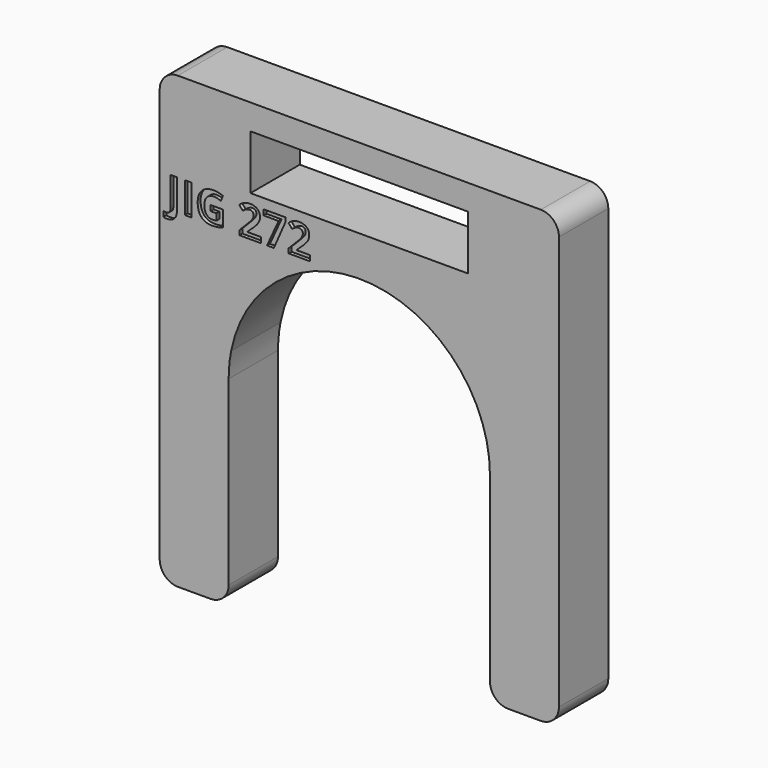
from build123d import *

# Parameters (mm, degrees)
F0_W     = 1.204434487
F0_H     = 8.486159523
F0_W_2   = 0.5953222601
F1_DEPTH = 17
F2_DEPTH = 5
F3_R     = 5
F4_DEPTH = 19
F5_DEPTH = 3


# Not quite as in the source:
# - a feature names something its author has since deleted; it is built from what else it names


with BuildPart() as f1:
    # F0 (on Front) → F1 (new body)
    with BuildSketch(Plane.XZ):
        with BuildLine():
            Line((0, 40), (0, 29))
            ThreePointArc((0, 29), (25.4558441227, 18.4558441227), (36, -7))
            Line((36, -7), (36, -62))
            Line((36, -62), (47.5, -62))
            Line((47.5, -62), (55, -62))
            Line((55, -62), (55, 0))
            Line((55, 0), (55, 62))
            Line((55, 62), (0, 62))
            Line((0, 62), (0, 55))
            Line((0, 55), (30, 55))
            Line((30, 55), (30, 40))
            Line((30, 40), (0, 40))
        make_face()
        with BuildLine():
            ThreePointArc((51, -33), (49.9748737342, -35.4748737342), (47.5, -36.5))
            ThreePointArc((47.5, -36.5), (44, -33), (47.5, -29.5))
            ThreePointArc((47.5, -29.5), (49.9748737342, -30.5251262658), (51, -33))
        make_face(mode=Mode.SUBTRACT)
        with BuildLine():
            ThreePointArc((50.5, 55), (49.6213203436, 52.8786796564), (47.5, 52))
            ThreePointArc((47.5, 52), (45.3786796564, 57.1213203436), (50.5, 55))
        make_face(mode=Mode.SUBTRACT)
        with BuildLine():
            Line((-36, 0), (-35.312887166, 0))
            ThreePointArc((-35.312887166, 0), (-22.8473193176, 20.8208554865), (0, 29))
            Line((0, 29), (0, 40))
            Line((0, 40), (-30, 40))
            Line((-30, 40), (-30, 55))
            Line((-30, 55), (0, 55))
            Line((0, 55), (0, 62))
            Line((0, 62), (-55, 62))
            Line((-55, 62), (-55, 0))
            Line((-55, 0), (-47.5, 0))
            Line((-47.5, 0), (-36, 0))
        make_face()
        with BuildLine():
            add(Edge.make_bspline(
                [(-50.9101120954, 27.0733917031), (-51.5889677105, 26.2951687134), (-52.9188189293, 26.2951687134)],
                knots=[0, 0, 0, 1, 1, 1], degree=2))
            add(Edge.make_bspline(
                [(-52.9188189293, 26.2951687134), (-53.5280245155, 26.2951687134), (-53.981214037, 26.4233247666)],
                knots=[0, 0, 0, 1, 1, 1], degree=2))
            Line((-53.981214037, 26.4233247666), (-53.981214037, 27.9203360547))
            add(Edge.make_bspline(
                [(-53.981214037, 27.9203360547), (-53.5168805109, 27.8051813402), (-53.1342696854, 27.8051813402)],
                knots=[0, 0, 0, 1, 1, 1], degree=2))
            add(Edge.make_bspline(
                [(-53.1342696854, 27.8051813402), (-52.5417801061, 27.8051813402), (-52.2863966667, 28.1738621599)],
                knots=[0, 0, 0, 1, 1, 1], degree=2))
            add(Edge.make_bspline(
                [(-52.2863966667, 28.1738621599), (-52.0310132274, 28.5425429797), (-52.0310132274, 29.3263379717)],
                knots=[0, 0, 0, 1, 1, 1], degree=2))
            Line((-52.0310132274, 29.3263379717), (-52.0310132274, 37.2775852726))
            Line((-52.0310132274, 37.2775852726), (-50.2312564802, 37.2775852726))
            Line((-50.2312564802, 37.2775852726), (-50.2312564802, 29.3374819764))
            add(Edge.make_bspline(
                [(-50.2312564802, 29.3374819764), (-50.2312564802, 27.8516146928), (-50.9101120954, 27.0733917031)],
                knots=[0, 0, 0, 1, 1, 1], degree=2))
        make_face(mode=Mode.SUBTRACT)
        Polygon((-46.295565513, 28.7914257497), (-47.5, 28.7914257497), (-48.0953222601, 28.7914257497), (-48.0953222601, 37.2775852726), (-47.5, 37.2775852726), (-46.295565513, 37.2775852726), align=None, mode=Mode.SUBTRACT)
        with BuildLine():
            Line((-40.9390139559, 32.0584764393), (-40.9390139559, 33.5573450615))
            Line((-40.9390139559, 33.5573450615), (-37.5716672247, 33.5573450615))
            Line((-37.5716672247, 33.5573450615), (-37.5716672247, 29.1573205682))
            add(Edge.make_bspline(
                [(-37.5716672247, 29.1573205682), (-38.3907515647, 28.8898644572), (-39.1132545313, 28.7821390791)],
                knots=[0, 0, 0, 1, 1, 1], degree=2))
            add(Edge.make_bspline(
                [(-39.1132545313, 28.7821390791), (-39.8357574979, 28.6744137011), (-40.5898351443, 28.6744137011)],
                knots=[0, 0, 0, 1, 1, 1], degree=2))
            add(Edge.make_bspline(
                [(-40.5898351443, 28.6744137011), (-42.5103186082, 28.6744137011), (-43.5234943622, 29.8036728366)],
                knots=[0, 0, 0, 1, 1, 1], degree=2))
            add(Edge.make_bspline(
                [(-43.5234943622, 29.8036728366), (-44.5366701161, 30.932931972), (-44.5366701161, 33.0465781828)],
                knots=[0, 0, 0, 1, 1, 1], degree=2))
            add(Edge.make_bspline(
                [(-44.5366701161, 33.0465781828), (-44.5366701161, 35.1007897023), (-43.3609776281, 36.2495508458)],
                knots=[0, 0, 0, 1, 1, 1], degree=2))
            add(Edge.make_bspline(
                [(-43.3609776281, 36.2495508458), (-42.18528514, 37.3983119894), (-40.1032136089, 37.3983119894)],
                knots=[0, 0, 0, 1, 1, 1], degree=2))
            add(Edge.make_bspline(
                [(-40.1032136089, 37.3983119894), (-38.7956503995, 37.3983119894), (-37.5828112293, 36.8764011061)],
                knots=[0, 0, 0, 1, 1, 1], degree=2))
            Line((-37.5828112293, 36.8764011061), (-38.1808728109, 35.4369671752))
            add(Edge.make_bspline(
                [(-38.1808728109, 35.4369671752), (-39.1095398631, 35.9013007013), (-40.1143576136, 35.9013007013)],
                knots=[0, 0, 0, 1, 1, 1], degree=2))
            add(Edge.make_bspline(
                [(-40.1143576136, 35.9013007013), (-41.2807634311, 35.9013007013), (-41.9828357226, 35.1175057092)],
                knots=[0, 0, 0, 1, 1, 1], degree=2))
            add(Edge.make_bspline(
                [(-41.9828357226, 35.1175057092), (-42.6849080141, 34.3337107172), (-42.6849080141, 33.0112888348)],
                knots=[0, 0, 0, 1, 1, 1], degree=2))
            add(Edge.make_bspline(
                [(-42.6849080141, 33.0112888348), (-42.6849080141, 31.6294322612), (-42.1193497793, 30.9013572922)],
                knots=[0, 0, 0, 1, 1, 1], degree=2))
            add(Edge.make_bspline(
                [(-42.1193497793, 30.9013572922), (-41.5537915445, 30.1732823233), (-40.4746804298, 30.1732823233)],
                knots=[0, 0, 0, 1, 1, 1], degree=2))
            add(Edge.make_bspline(
                [(-40.4746804298, 30.1732823233), (-39.9100508621, 30.1732823233), (-39.3305626215, 30.2884370378)],
                knots=[0, 0, 0, 1, 1, 1], degree=2))
            Line((-39.3305626215, 30.2884370378), (-39.3305626215, 32.0584764393))
            Line((-39.3305626215, 32.0584764393), (-40.9390139559, 32.0584764393))
        make_face(mode=Mode.SUBTRACT)
        with BuildLine():
            Line((-27.1241628875, 30.3014383765), (-27.1241628875, 28.7914257497))
            Line((-27.1241628875, 28.7914257497), (-33.0564880169, 28.7914257497))
            Line((-33.0564880169, 28.7914257497), (-33.0564880169, 30.0395542678))
            Line((-33.0564880169, 30.0395542678), (-30.9261257991, 32.1922044948))
            add(Edge.make_bspline(
                [(-30.9261257991, 32.1922044948), (-29.9788854059, 33.1617328973), (-29.6891412856, 33.5359857193)],
                knots=[0, 0, 0, 1, 1, 1], degree=2))
            add(Edge.make_bspline(
                [(-29.6891412856, 33.5359857193), (-29.3993971653, 33.9102385414), (-29.2712411121, 34.2297000073)],
                knots=[0, 0, 0, 1, 1, 1], degree=2))
            add(Edge.make_bspline(
                [(-29.2712411121, 34.2297000073), (-29.1430850589, 34.5491614733), (-29.1430850589, 34.8909109485)],
                knots=[0, 0, 0, 1, 1, 1], degree=2))
            add(Edge.make_bspline(
                [(-29.1430850589, 34.8909109485), (-29.1430850589, 35.4016778272), (-29.4253998428, 35.6514892642)],
                knots=[0, 0, 0, 1, 1, 1], degree=2))
            add(Edge.make_bspline(
                [(-29.4253998428, 35.6514892642), (-29.7077146267, 35.9013007013), (-30.1776201551, 35.9013007013)],
                knots=[0, 0, 0, 1, 1, 1], degree=2))
            add(Edge.make_bspline(
                [(-30.1776201551, 35.9013007013), (-30.6698136927, 35.9013007013), (-31.1341472188, 35.6747059405)],
                knots=[0, 0, 0, 1, 1, 1], degree=2))
            add(Edge.make_bspline(
                [(-31.1341472188, 35.6747059405), (-31.5984807449, 35.4481111798), (-32.1036756213, 35.0302110063)],
                knots=[0, 0, 0, 1, 1, 1], degree=2))
            Line((-32.1036756213, 35.0302110063), (-33.0787760261, 36.1854728192))
            add(Edge.make_bspline(
                [(-33.0787760261, 36.1854728192), (-32.452854433, 36.7203850413), (-32.0405262618, 36.9404791327)],
                knots=[0, 0, 0, 1, 1, 1], degree=2))
            add(Edge.make_bspline(
                [(-32.0405262618, 36.9404791327), (-31.6281980906, 37.1605732241), (-31.1406478882, 37.2794426067)],
                knots=[0, 0, 0, 1, 1, 1], degree=2))
            add(Edge.make_bspline(
                [(-31.1406478882, 37.2794426067), (-30.6530976858, 37.3983119894), (-30.0494641019, 37.3983119894)],
                knots=[0, 0, 0, 1, 1, 1], degree=2))
            add(Edge.make_bspline(
                [(-30.0494641019, 37.3983119894), (-29.2545251052, 37.3983119894), (-28.645319519, 37.1085678691)],
                knots=[0, 0, 0, 1, 1, 1], degree=2))
            add(Edge.make_bspline(
                [(-28.645319519, 37.1085678691), (-28.0361139327, 36.8188237488), (-27.6990077928, 36.2959841985)],
                knots=[0, 0, 0, 1, 1, 1], degree=2))
            add(Edge.make_bspline(
                [(-27.6990077928, 36.2959841985), (-27.3619016528, 35.7731446481), (-27.3619016528, 35.1007897023)],
                knots=[0, 0, 0, 1, 1, 1], degree=2))
            add(Edge.make_bspline(
                [(-27.3619016528, 35.1007897023), (-27.3619016528, 34.5138721253), (-27.5680657384, 34.0003192454)],
                knots=[0, 0, 0, 1, 1, 1], degree=2))
            add(Edge.make_bspline(
                [(-27.5680657384, 34.0003192454), (-27.774229824, 33.4867663656), (-28.2069886703, 32.9472108082)],
                knots=[0, 0, 0, 1, 1, 1], degree=2))
            add(Edge.make_bspline(
                [(-28.2069886703, 32.9472108082), (-28.6397475166, 32.4076552509), (-29.7300026359, 31.4084095027)],
                knots=[0, 0, 0, 1, 1, 1], degree=2))
            Line((-29.7300026359, 31.4084095027), (-30.8221150893, 30.381303743))
            Line((-30.8221150893, 30.381303743), (-30.8221150893, 30.3014383765))
            Line((-30.8221150893, 30.3014383765), (-27.1241628875, 30.3014383765))
        make_face(mode=Mode.SUBTRACT)
        with BuildLine():
            ThreePointArc((-44.5, 55), (-45.3786796564, 52.8786796564), (-47.5, 52))
            ThreePointArc((-47.5, 52), (-49.6213203436, 57.1213203436), (-44.5, 55))
        make_face(mode=Mode.SUBTRACT)
        Polygon((-23.5487947365, 28.7914257497), (-25.4302741842, 28.7914257497), (-22.2430888611, 35.7564286411), (-26.4276625983, 35.7564286411), (-26.4276625983, 37.266441268), (-20.3393214041, 37.266441268), (-20.3393214041, 36.1390394666), align=None, mode=Mode.SUBTRACT)
        with BuildLine():
            Line((-13.5544799208, 30.3014383765), (-13.5544799208, 28.7914257497))
            Line((-13.5544799208, 28.7914257497), (-19.4868050502, 28.7914257497))
            Line((-19.4868050502, 28.7914257497), (-19.4868050502, 30.0395542678))
            Line((-19.4868050502, 30.0395542678), (-17.3564428325, 32.1922044948))
            add(Edge.make_bspline(
                [(-17.3564428325, 32.1922044948), (-16.4092024392, 33.1617328973), (-16.1194583189, 33.5359857193)],
                knots=[0, 0, 0, 1, 1, 1], degree=2))
            add(Edge.make_bspline(
                [(-16.1194583189, 33.5359857193), (-15.8297141986, 33.9102385414), (-15.7015581454, 34.2297000073)],
                knots=[0, 0, 0, 1, 1, 1], degree=2))
            add(Edge.make_bspline(
                [(-15.7015581454, 34.2297000073), (-15.5734020922, 34.5491614733), (-15.5734020922, 34.8909109485)],
                knots=[0, 0, 0, 1, 1, 1], degree=2))
            add(Edge.make_bspline(
                [(-15.5734020922, 34.8909109485), (-15.5734020922, 35.4016778272), (-15.8557168761, 35.6514892642)],
                knots=[0, 0, 0, 1, 1, 1], degree=2))
            add(Edge.make_bspline(
                [(-15.8557168761, 35.6514892642), (-16.13803166, 35.9013007013), (-16.6079371884, 35.9013007013)],
                knots=[0, 0, 0, 1, 1, 1], degree=2))
            add(Edge.make_bspline(
                [(-16.6079371884, 35.9013007013), (-17.100130726, 35.9013007013), (-17.5644642521, 35.6747059405)],
                knots=[0, 0, 0, 1, 1, 1], degree=2))
            add(Edge.make_bspline(
                [(-17.5644642521, 35.6747059405), (-18.0287977782, 35.4481111798), (-18.5339926546, 35.0302110063)],
                knots=[0, 0, 0, 1, 1, 1], degree=2))
            Line((-18.5339926546, 35.0302110063), (-19.5090930594, 36.1854728192))
            add(Edge.make_bspline(
                [(-19.5090930594, 36.1854728192), (-18.8831714663, 36.7203850413), (-18.4708432951, 36.9404791327)],
                knots=[0, 0, 0, 1, 1, 1], degree=2))
            add(Edge.make_bspline(
                [(-18.4708432951, 36.9404791327), (-18.0585151239, 37.1605732241), (-17.5709649215, 37.2794426067)],
                knots=[0, 0, 0, 1, 1, 1], degree=2))
            add(Edge.make_bspline(
                [(-17.5709649215, 37.2794426067), (-17.0834147191, 37.3983119894), (-16.4797811352, 37.3983119894)],
                knots=[0, 0, 0, 1, 1, 1], degree=2))
            add(Edge.make_bspline(
                [(-16.4797811352, 37.3983119894), (-15.6848421385, 37.3983119894), (-15.0756365523, 37.1085678691)],
                knots=[0, 0, 0, 1, 1, 1], degree=2))
            add(Edge.make_bspline(
                [(-15.0756365523, 37.1085678691), (-14.466430966, 36.8188237488), (-14.1293248261, 36.2959841985)],
                knots=[0, 0, 0, 1, 1, 1], degree=2))
            add(Edge.make_bspline(
                [(-14.1293248261, 36.2959841985), (-13.7922186861, 35.7731446481), (-13.7922186861, 35.1007897023)],
                knots=[0, 0, 0, 1, 1, 1], degree=2))
            add(Edge.make_bspline(
                [(-13.7922186861, 35.1007897023), (-13.7922186861, 34.5138721253), (-13.9983827717, 34.0003192454)],
                knots=[0, 0, 0, 1, 1, 1], degree=2))
            add(Edge.make_bspline(
                [(-13.9983827717, 34.0003192454), (-14.2045468573, 33.4867663656), (-14.6373057036, 32.9472108082)],
                knots=[0, 0, 0, 1, 1, 1], degree=2))
            add(Edge.make_bspline(
                [(-14.6373057036, 32.9472108082), (-15.0700645499, 32.4076552509), (-16.1603196692, 31.4084095027)],
                knots=[0, 0, 0, 1, 1, 1], degree=2))
            Line((-16.1603196692, 31.4084095027), (-17.2524321226, 30.381303743))
            Line((-17.2524321226, 30.381303743), (-17.2524321226, 30.3014383765))
            Line((-17.2524321226, 30.3014383765), (-13.5544799208, 30.3014383765))
        make_face(mode=Mode.SUBTRACT)
        with BuildLine():
            Line((-36, -7), (-36, 0))
            Line((-36, 0), (-47.5, 0))
            Line((-47.5, 0), (-47.5, -29.5))
            ThreePointArc((-47.5, -29.5), (-45.0251262658, -30.5251262658), (-44, -33))
            ThreePointArc((-44, -33), (-45.0251262658, -35.4748737342), (-47.5, -36.5))
            Line((-47.5, -36.5), (-47.5, -62))
            Line((-47.5, -62), (-36, -62))
            Line((-36, -62), (-36, -7))
        make_face()
        with BuildLine():
            Line((-47.5, -29.5), (-47.5, 0))
            Line((-47.5, 0), (-55, 0))
            Line((-55, 0), (-55, -62))
            Line((-55, -62), (-47.5, -62))
            Line((-47.5, -62), (-47.5, -36.5))
            ThreePointArc((-47.5, -36.5), (-51, -33), (-47.5, -29.5))
        make_face()
        with BuildLine():
            Line((-37.5716672247, 33.5573450615), (-40.9390139559, 33.5573450615))
            Line((-40.9390139559, 33.5573450615), (-40.9390139559, 32.0584764393))
            Line((-40.9390139559, 32.0584764393), (-39.3305626215, 32.0584764393))
            Line((-39.3305626215, 32.0584764393), (-39.3305626215, 30.2884370378))
            add(Edge.make_bspline(
                [(-40.4746804298, 30.1732823233), (-39.9100508621, 30.1732823233), (-39.3305626215, 30.2884370378)],
                knots=[0, 0, 0, 1, 1, 1], degree=2))
            add(Edge.make_bspline(
                [(-42.1193497793, 30.9013572922), (-41.5537915445, 30.1732823233), (-40.4746804298, 30.1732823233)],
                knots=[0, 0, 0, 1, 1, 1], degree=2))
            add(Edge.make_bspline(
                [(-42.6849080141, 33.0112888348), (-42.6849080141, 31.6294322612), (-42.1193497793, 30.9013572922)],
                knots=[0, 0, 0, 1, 1, 1], degree=2))
            add(Edge.make_bspline(
                [(-41.9828357226, 35.1175057092), (-42.6849080141, 34.3337107172), (-42.6849080141, 33.0112888348)],
                knots=[0, 0, 0, 1, 1, 1], degree=2))
            add(Edge.make_bspline(
                [(-40.1143576136, 35.9013007013), (-41.2807634311, 35.9013007013), (-41.9828357226, 35.1175057092)],
                knots=[0, 0, 0, 1, 1, 1], degree=2))
            add(Edge.make_bspline(
                [(-38.1808728109, 35.4369671752), (-39.1095398631, 35.9013007013), (-40.1143576136, 35.9013007013)],
                knots=[0, 0, 0, 1, 1, 1], degree=2))
            Line((-38.1808728109, 35.4369671752), (-37.5828112293, 36.8764011061))
            add(Edge.make_bspline(
                [(-40.1032136089, 37.3983119894), (-38.7956503995, 37.3983119894), (-37.5828112293, 36.8764011061)],
                knots=[0, 0, 0, 1, 1, 1], degree=2))
            add(Edge.make_bspline(
                [(-43.3609776281, 36.2495508458), (-42.18528514, 37.3983119894), (-40.1032136089, 37.3983119894)],
                knots=[0, 0, 0, 1, 1, 1], degree=2))
            add(Edge.make_bspline(
                [(-44.5366701161, 33.0465781828), (-44.5366701161, 35.1007897023), (-43.3609776281, 36.2495508458)],
                knots=[0, 0, 0, 1, 1, 1], degree=2))
            add(Edge.make_bspline(
                [(-43.5234943622, 29.8036728366), (-44.5366701161, 30.932931972), (-44.5366701161, 33.0465781828)],
                knots=[0, 0, 0, 1, 1, 1], degree=2))
            add(Edge.make_bspline(
                [(-40.5898351443, 28.6744137011), (-42.5103186082, 28.6744137011), (-43.5234943622, 29.8036728366)],
                knots=[0, 0, 0, 1, 1, 1], degree=2))
            add(Edge.make_bspline(
                [(-39.1132545313, 28.7821390791), (-39.8357574979, 28.6744137011), (-40.5898351443, 28.6744137011)],
                knots=[0, 0, 0, 1, 1, 1], degree=2))
            add(Edge.make_bspline(
                [(-37.5716672247, 29.1573205682), (-38.3907515647, 28.8898644572), (-39.1132545313, 28.7821390791)],
                knots=[0, 0, 0, 1, 1, 1], degree=2))
            Line((-37.5716672247, 29.1573205682), (-37.5716672247, 33.5573450615))
        make_face()
        with BuildLine():
            ThreePointArc((-44.5, 55), (-49.6213203436, 57.1213203436), (-47.5, 52))
            ThreePointArc((-47.5, 52), (-45.3786796564, 52.8786796564), (-44.5, 55))
        make_face()
        with BuildLine():
            ThreePointArc((50.5, 55), (45.3786796564, 57.1213203436), (47.5, 52))
            ThreePointArc((47.5, 52), (49.6213203436, 52.8786796564), (50.5, 55))
        make_face()
        with BuildLine():
            Line((-33.0564880169, 28.7914257497), (-27.1241628875, 28.7914257497))
            Line((-27.1241628875, 28.7914257497), (-27.1241628875, 30.3014383765))
            Line((-27.1241628875, 30.3014383765), (-30.8221150893, 30.3014383765))
            Line((-30.8221150893, 30.3014383765), (-30.8221150893, 30.381303743))
            Line((-30.8221150893, 30.381303743), (-29.7300026359, 31.4084095027))
            add(Edge.make_bspline(
                [(-28.2069886703, 32.9472108082), (-28.6397475166, 32.4076552509), (-29.7300026359, 31.4084095027)],
                knots=[0, 0, 0, 1, 1, 1], degree=2))
            add(Edge.make_bspline(
                [(-27.5680657384, 34.0003192454), (-27.774229824, 33.4867663656), (-28.2069886703, 32.9472108082)],
                knots=[0, 0, 0, 1, 1, 1], degree=2))
            add(Edge.make_bspline(
                [(-27.3619016528, 35.1007897023), (-27.3619016528, 34.5138721253), (-27.5680657384, 34.0003192454)],
                knots=[0, 0, 0, 1, 1, 1], degree=2))
            add(Edge.make_bspline(
                [(-27.6990077928, 36.2959841985), (-27.3619016528, 35.7731446481), (-27.3619016528, 35.1007897023)],
                knots=[0, 0, 0, 1, 1, 1], degree=2))
            add(Edge.make_bspline(
                [(-28.645319519, 37.1085678691), (-28.0361139327, 36.8188237488), (-27.6990077928, 36.2959841985)],
                knots=[0, 0, 0, 1, 1, 1], degree=2))
            add(Edge.make_bspline(
                [(-30.0494641019, 37.3983119894), (-29.2545251052, 37.3983119894), (-28.645319519, 37.1085678691)],
                knots=[0, 0, 0, 1, 1, 1], degree=2))
            add(Edge.make_bspline(
                [(-31.1406478882, 37.2794426067), (-30.6530976858, 37.3983119894), (-30.0494641019, 37.3983119894)],
                knots=[0, 0, 0, 1, 1, 1], degree=2))
            add(Edge.make_bspline(
                [(-32.0405262618, 36.9404791327), (-31.6281980906, 37.1605732241), (-31.1406478882, 37.2794426067)],
                knots=[0, 0, 0, 1, 1, 1], degree=2))
            add(Edge.make_bspline(
                [(-33.0787760261, 36.1854728192), (-32.452854433, 36.7203850413), (-32.0405262618, 36.9404791327)],
                knots=[0, 0, 0, 1, 1, 1], degree=2))
            Line((-33.0787760261, 36.1854728192), (-32.1036756213, 35.0302110063))
            add(Edge.make_bspline(
                [(-31.1341472188, 35.6747059405), (-31.5984807449, 35.4481111798), (-32.1036756213, 35.0302110063)],
                knots=[0, 0, 0, 1, 1, 1], degree=2))
            add(Edge.make_bspline(
                [(-30.1776201551, 35.9013007013), (-30.6698136927, 35.9013007013), (-31.1341472188, 35.6747059405)],
                knots=[0, 0, 0, 1, 1, 1], degree=2))
            add(Edge.make_bspline(
                [(-29.4253998428, 35.6514892642), (-29.7077146267, 35.9013007013), (-30.1776201551, 35.9013007013)],
                knots=[0, 0, 0, 1, 1, 1], degree=2))
            add(Edge.make_bspline(
                [(-29.1430850589, 34.8909109485), (-29.1430850589, 35.4016778272), (-29.4253998428, 35.6514892642)],
                knots=[0, 0, 0, 1, 1, 1], degree=2))
            add(Edge.make_bspline(
                [(-29.2712411121, 34.2297000073), (-29.1430850589, 34.5491614733), (-29.1430850589, 34.8909109485)],
                knots=[0, 0, 0, 1, 1, 1], degree=2))
            add(Edge.make_bspline(
                [(-29.6891412856, 33.5359857193), (-29.3993971653, 33.9102385414), (-29.2712411121, 34.2297000073)],
                knots=[0, 0, 0, 1, 1, 1], degree=2))
            add(Edge.make_bspline(
                [(-30.9261257991, 32.1922044948), (-29.9788854059, 33.1617328973), (-29.6891412856, 33.5359857193)],
                knots=[0, 0, 0, 1, 1, 1], degree=2))
            Line((-30.9261257991, 32.1922044948), (-33.0564880169, 30.0395542678))
            Line((-33.0564880169, 30.0395542678), (-33.0564880169, 28.7914257497))
        make_face()
        with BuildLine():
            Line((-19.4868050502, 28.7914257497), (-13.5544799208, 28.7914257497))
            Line((-13.5544799208, 28.7914257497), (-13.5544799208, 30.3014383765))
            Line((-13.5544799208, 30.3014383765), (-17.2524321226, 30.3014383765))
            Line((-17.2524321226, 30.3014383765), (-17.2524321226, 30.381303743))
            Line((-17.2524321226, 30.381303743), (-16.1603196692, 31.4084095027))
            add(Edge.make_bspline(
                [(-14.6373057036, 32.9472108082), (-15.0700645499, 32.4076552509), (-16.1603196692, 31.4084095027)],
                knots=[0, 0, 0, 1, 1, 1], degree=2))
            add(Edge.make_bspline(
                [(-13.9983827717, 34.0003192454), (-14.2045468573, 33.4867663656), (-14.6373057036, 32.9472108082)],
                knots=[0, 0, 0, 1, 1, 1], degree=2))
            add(Edge.make_bspline(
                [(-13.7922186861, 35.1007897023), (-13.7922186861, 34.5138721253), (-13.9983827717, 34.0003192454)],
                knots=[0, 0, 0, 1, 1, 1], degree=2))
            add(Edge.make_bspline(
                [(-14.1293248261, 36.2959841985), (-13.7922186861, 35.7731446481), (-13.7922186861, 35.1007897023)],
                knots=[0, 0, 0, 1, 1, 1], degree=2))
            add(Edge.make_bspline(
                [(-15.0756365523, 37.1085678691), (-14.466430966, 36.8188237488), (-14.1293248261, 36.2959841985)],
                knots=[0, 0, 0, 1, 1, 1], degree=2))
            add(Edge.make_bspline(
                [(-16.4797811352, 37.3983119894), (-15.6848421385, 37.3983119894), (-15.0756365523, 37.1085678691)],
                knots=[0, 0, 0, 1, 1, 1], degree=2))
            add(Edge.make_bspline(
                [(-17.5709649215, 37.2794426067), (-17.0834147191, 37.3983119894), (-16.4797811352, 37.3983119894)],
                knots=[0, 0, 0, 1, 1, 1], degree=2))
            add(Edge.make_bspline(
                [(-18.4708432951, 36.9404791327), (-18.0585151239, 37.1605732241), (-17.5709649215, 37.2794426067)],
                knots=[0, 0, 0, 1, 1, 1], degree=2))
            add(Edge.make_bspline(
                [(-19.5090930594, 36.1854728192), (-18.8831714663, 36.7203850413), (-18.4708432951, 36.9404791327)],
                knots=[0, 0, 0, 1, 1, 1], degree=2))
            Line((-19.5090930594, 36.1854728192), (-18.5339926546, 35.0302110063))
            add(Edge.make_bspline(
                [(-17.5644642521, 35.6747059405), (-18.0287977782, 35.4481111798), (-18.5339926546, 35.0302110063)],
                knots=[0, 0, 0, 1, 1, 1], degree=2))
            add(Edge.make_bspline(
                [(-16.6079371884, 35.9013007013), (-17.100130726, 35.9013007013), (-17.5644642521, 35.6747059405)],
                knots=[0, 0, 0, 1, 1, 1], degree=2))
            add(Edge.make_bspline(
                [(-15.8557168761, 35.6514892642), (-16.13803166, 35.9013007013), (-16.6079371884, 35.9013007013)],
                knots=[0, 0, 0, 1, 1, 1], degree=2))
            add(Edge.make_bspline(
                [(-15.5734020922, 34.8909109485), (-15.5734020922, 35.4016778272), (-15.8557168761, 35.6514892642)],
                knots=[0, 0, 0, 1, 1, 1], degree=2))
            add(Edge.make_bspline(
                [(-15.7015581454, 34.2297000073), (-15.5734020922, 34.5491614733), (-15.5734020922, 34.8909109485)],
                knots=[0, 0, 0, 1, 1, 1], degree=2))
            add(Edge.make_bspline(
                [(-16.1194583189, 33.5359857193), (-15.8297141986, 33.9102385414), (-15.7015581454, 34.2297000073)],
                knots=[0, 0, 0, 1, 1, 1], degree=2))
            add(Edge.make_bspline(
                [(-17.3564428325, 32.1922044948), (-16.4092024392, 33.1617328973), (-16.1194583189, 33.5359857193)],
                knots=[0, 0, 0, 1, 1, 1], degree=2))
            Line((-17.3564428325, 32.1922044948), (-19.4868050502, 30.0395542678))
            Line((-19.4868050502, 30.0395542678), (-19.4868050502, 28.7914257497))
        make_face()
        Polygon((-22.2430888611, 35.7564286411), (-25.4302741842, 28.7914257497), (-23.5487947365, 28.7914257497), (-20.3393214041, 36.1390394666), (-20.3393214041, 37.266441268), (-26.4276625983, 37.266441268), (-26.4276625983, 35.7564286411), align=None)
        with BuildLine():
            add(Edge.make_bspline(
                [(-52.9188189293, 26.2951687134), (-53.5280245155, 26.2951687134), (-53.981214037, 26.4233247666)],
                knots=[0, 0, 0, 1, 1, 1], degree=2))
            add(Edge.make_bspline(
                [(-50.9101120954, 27.0733917031), (-51.5889677105, 26.2951687134), (-52.9188189293, 26.2951687134)],
                knots=[0, 0, 0, 1, 1, 1], degree=2))
            add(Edge.make_bspline(
                [(-50.2312564802, 29.3374819764), (-50.2312564802, 27.8516146928), (-50.9101120954, 27.0733917031)],
                knots=[0, 0, 0, 1, 1, 1], degree=2))
            Line((-50.2312564802, 29.3374819764), (-50.2312564802, 37.2775852726))
            Line((-50.2312564802, 37.2775852726), (-52.0310132274, 37.2775852726))
            Line((-52.0310132274, 37.2775852726), (-52.0310132274, 29.3263379717))
            add(Edge.make_bspline(
                [(-52.2863966667, 28.1738621599), (-52.0310132274, 28.5425429797), (-52.0310132274, 29.3263379717)],
                knots=[0, 0, 0, 1, 1, 1], degree=2))
            add(Edge.make_bspline(
                [(-53.1342696854, 27.8051813402), (-52.5417801061, 27.8051813402), (-52.2863966667, 28.1738621599)],
                knots=[0, 0, 0, 1, 1, 1], degree=2))
            add(Edge.make_bspline(
                [(-53.981214037, 27.9203360547), (-53.5168805109, 27.8051813402), (-53.1342696854, 27.8051813402)],
                knots=[0, 0, 0, 1, 1, 1], degree=2))
            Line((-53.981214037, 27.9203360547), (-53.981214037, 26.4233247666))
        make_face()
        with BuildLine():
            ThreePointArc((-44, -33), (-45.0251262658, -30.5251262658), (-47.5, -29.5))
            Line((-47.5, -29.5), (-47.5, -33))
            Line((-47.5, -33), (-47.5, -36.5))
            ThreePointArc((-47.5, -36.5), (-45.0251262658, -35.4748737342), (-44, -33))
        make_face()
        with BuildLine():
            Line((-47.5, -33), (-47.5, -29.5))
            ThreePointArc((-47.5, -29.5), (-51, -33), (-47.5, -36.5))
            Line((-47.5, -36.5), (-47.5, -33))
        make_face()
        with BuildLine():
            ThreePointArc((47.5, -29.5), (44, -33), (47.5, -36.5))
            Line((47.5, -36.5), (47.5, -33))
            Line((47.5, -33), (47.5, -29.5))
        make_face()
        with BuildLine():
            Line((47.5, -33), (47.5, -36.5))
            ThreePointArc((47.5, -36.5), (49.9748737342, -35.4748737342), (51, -33))
            ThreePointArc((51, -33), (49.9748737342, -30.5251262658), (47.5, -29.5))
            Line((47.5, -29.5), (47.5, -33))
        make_face()
        with Locations((-46.8977827565, 33.0345055111)):
            Rectangle(F0_W, F0_H)
        with Locations((-47.7976611301, 33.0345055111)):
            Rectangle(F0_W_2, F0_H)
        with BuildLine():
            ThreePointArc((-36, -7), (-35.8278099943, -3.4831788485), (-35.312887166, 0))
            Line((-35.312887166, 0), (-36, 0))
            Line((-36, 0), (-36, -7))
        make_face()
    extrude(amount=F1_DEPTH)

    # F0 (on Front) → F2 (join)
    with BuildSketch(Plane.XZ):
        with BuildLine():
            ThreePointArc((-44.5, 55), (-49.6213203436, 57.1213203436), (-47.5, 52))
            ThreePointArc((-47.5, 52), (-45.3786796564, 52.8786796564), (-44.5, 55))
        make_face()
        with BuildLine():
            Line((-47.5, -33), (-47.5, -29.5))
            ThreePointArc((-47.5, -29.5), (-51, -33), (-47.5, -36.5))
            Line((-47.5, -36.5), (-47.5, -33))
        make_face()
        with BuildLine():
            ThreePointArc((-44, -33), (-45.0251262658, -30.5251262658), (-47.5, -29.5))
            Line((-47.5, -29.5), (-47.5, -33))
            Line((-47.5, -33), (-47.5, -36.5))
            ThreePointArc((-47.5, -36.5), (-45.0251262658, -35.4748737342), (-44, -33))
        make_face()
        with BuildLine():
            ThreePointArc((50.5, 55), (45.3786796564, 57.1213203436), (47.5, 52))
            ThreePointArc((47.5, 52), (49.6213203436, 52.8786796564), (50.5, 55))
        make_face()
        with BuildLine():
            ThreePointArc((47.5, -29.5), (44, -33), (47.5, -36.5))
            Line((47.5, -36.5), (47.5, -33))
            Line((47.5, -33), (47.5, -29.5))
        make_face()
        with BuildLine():
            Line((47.5, -33), (47.5, -36.5))
            ThreePointArc((47.5, -36.5), (49.9748737342, -35.4748737342), (51, -33))
            ThreePointArc((51, -33), (49.9748737342, -30.5251262658), (47.5, -29.5))
            Line((47.5, -29.5), (47.5, -33))
        make_face()
    extrude(amount=-F2_DEPTH)

    # F3
    f3_edges = [f1.edges().sort_by_distance(p)[0] for p in [
        (-55, -8.5, 62),
        (55, -8.5, 62),
        (-55, -8.5, -62),
        (-36, -8.5, -62),
        (36, -8.5, -62),
        (55, -8.5, -62),
    ]]
    fillet(f3_edges, radius=F3_R)

    # F0 (on Front) → F4 (join)
    with BuildSketch(Plane.XZ):
        with BuildLine():
            add(Edge.make_bspline(
                [(-52.9188189293, 26.2951687134), (-53.5280245155, 26.2951687134), (-53.981214037, 26.4233247666)],
                knots=[0, 0, 0, 1, 1, 1], degree=2))
            add(Edge.make_bspline(
                [(-50.9101120954, 27.0733917031), (-51.5889677105, 26.2951687134), (-52.9188189293, 26.2951687134)],
                knots=[0, 0, 0, 1, 1, 1], degree=2))
            add(Edge.make_bspline(
                [(-50.2312564802, 29.3374819764), (-50.2312564802, 27.8516146928), (-50.9101120954, 27.0733917031)],
                knots=[0, 0, 0, 1, 1, 1], degree=2))
            Line((-50.2312564802, 29.3374819764), (-50.2312564802, 37.2775852726))
            Line((-50.2312564802, 37.2775852726), (-52.0310132274, 37.2775852726))
            Line((-52.0310132274, 37.2775852726), (-52.0310132274, 29.3263379717))
            add(Edge.make_bspline(
                [(-52.2863966667, 28.1738621599), (-52.0310132274, 28.5425429797), (-52.0310132274, 29.3263379717)],
                knots=[0, 0, 0, 1, 1, 1], degree=2))
            add(Edge.make_bspline(
                [(-53.1342696854, 27.8051813402), (-52.5417801061, 27.8051813402), (-52.2863966667, 28.1738621599)],
                knots=[0, 0, 0, 1, 1, 1], degree=2))
            add(Edge.make_bspline(
                [(-53.981214037, 27.9203360547), (-53.5168805109, 27.8051813402), (-53.1342696854, 27.8051813402)],
                knots=[0, 0, 0, 1, 1, 1], degree=2))
            Line((-53.981214037, 27.9203360547), (-53.981214037, 26.4233247666))
        make_face()
        with Locations((-47.7976611301, 33.0345055111)):
            Rectangle(F0_W_2, F0_H)
        with Locations((-46.8977827565, 33.0345055111)):
            Rectangle(F0_W, F0_H)
        with BuildLine():
            Line((-37.5716672247, 33.5573450615), (-40.9390139559, 33.5573450615))
            Line((-40.9390139559, 33.5573450615), (-40.9390139559, 32.0584764393))
            Line((-40.9390139559, 32.0584764393), (-39.3305626215, 32.0584764393))
            Line((-39.3305626215, 32.0584764393), (-39.3305626215, 30.2884370378))
            add(Edge.make_bspline(
                [(-40.4746804298, 30.1732823233), (-39.9100508621, 30.1732823233), (-39.3305626215, 30.2884370378)],
                knots=[0, 0, 0, 1, 1, 1], degree=2))
            add(Edge.make_bspline(
                [(-42.1193497793, 30.9013572922), (-41.5537915445, 30.1732823233), (-40.4746804298, 30.1732823233)],
                knots=[0, 0, 0, 1, 1, 1], degree=2))
            add(Edge.make_bspline(
                [(-42.6849080141, 33.0112888348), (-42.6849080141, 31.6294322612), (-42.1193497793, 30.9013572922)],
                knots=[0, 0, 0, 1, 1, 1], degree=2))
            add(Edge.make_bspline(
                [(-41.9828357226, 35.1175057092), (-42.6849080141, 34.3337107172), (-42.6849080141, 33.0112888348)],
                knots=[0, 0, 0, 1, 1, 1], degree=2))
            add(Edge.make_bspline(
                [(-40.1143576136, 35.9013007013), (-41.2807634311, 35.9013007013), (-41.9828357226, 35.1175057092)],
                knots=[0, 0, 0, 1, 1, 1], degree=2))
            add(Edge.make_bspline(
                [(-38.1808728109, 35.4369671752), (-39.1095398631, 35.9013007013), (-40.1143576136, 35.9013007013)],
                knots=[0, 0, 0, 1, 1, 1], degree=2))
            Line((-38.1808728109, 35.4369671752), (-37.5828112293, 36.8764011061))
            add(Edge.make_bspline(
                [(-40.1032136089, 37.3983119894), (-38.7956503995, 37.3983119894), (-37.5828112293, 36.8764011061)],
                knots=[0, 0, 0, 1, 1, 1], degree=2))
            add(Edge.make_bspline(
                [(-43.3609776281, 36.2495508458), (-42.18528514, 37.3983119894), (-40.1032136089, 37.3983119894)],
                knots=[0, 0, 0, 1, 1, 1], degree=2))
            add(Edge.make_bspline(
                [(-44.5366701161, 33.0465781828), (-44.5366701161, 35.1007897023), (-43.3609776281, 36.2495508458)],
                knots=[0, 0, 0, 1, 1, 1], degree=2))
            add(Edge.make_bspline(
                [(-43.5234943622, 29.8036728366), (-44.5366701161, 30.932931972), (-44.5366701161, 33.0465781828)],
                knots=[0, 0, 0, 1, 1, 1], degree=2))
            add(Edge.make_bspline(
                [(-40.5898351443, 28.6744137011), (-42.5103186082, 28.6744137011), (-43.5234943622, 29.8036728366)],
                knots=[0, 0, 0, 1, 1, 1], degree=2))
            add(Edge.make_bspline(
                [(-39.1132545313, 28.7821390791), (-39.8357574979, 28.6744137011), (-40.5898351443, 28.6744137011)],
                knots=[0, 0, 0, 1, 1, 1], degree=2))
            add(Edge.make_bspline(
                [(-37.5716672247, 29.1573205682), (-38.3907515647, 28.8898644572), (-39.1132545313, 28.7821390791)],
                knots=[0, 0, 0, 1, 1, 1], degree=2))
            Line((-37.5716672247, 29.1573205682), (-37.5716672247, 33.5573450615))
        make_face()
        with BuildLine():
            Line((-33.0564880169, 28.7914257497), (-27.1241628875, 28.7914257497))
            Line((-27.1241628875, 28.7914257497), (-27.1241628875, 30.3014383765))
            Line((-27.1241628875, 30.3014383765), (-30.8221150893, 30.3014383765))
            Line((-30.8221150893, 30.3014383765), (-30.8221150893, 30.381303743))
            Line((-30.8221150893, 30.381303743), (-29.7300026359, 31.4084095027))
            add(Edge.make_bspline(
                [(-28.2069886703, 32.9472108082), (-28.6397475166, 32.4076552509), (-29.7300026359, 31.4084095027)],
                knots=[0, 0, 0, 1, 1, 1], degree=2))
            add(Edge.make_bspline(
                [(-27.5680657384, 34.0003192454), (-27.774229824, 33.4867663656), (-28.2069886703, 32.9472108082)],
                knots=[0, 0, 0, 1, 1, 1], degree=2))
            add(Edge.make_bspline(
                [(-27.3619016528, 35.1007897023), (-27.3619016528, 34.5138721253), (-27.5680657384, 34.0003192454)],
                knots=[0, 0, 0, 1, 1, 1], degree=2))
            add(Edge.make_bspline(
                [(-27.6990077928, 36.2959841985), (-27.3619016528, 35.7731446481), (-27.3619016528, 35.1007897023)],
                knots=[0, 0, 0, 1, 1, 1], degree=2))
            add(Edge.make_bspline(
                [(-28.645319519, 37.1085678691), (-28.0361139327, 36.8188237488), (-27.6990077928, 36.2959841985)],
                knots=[0, 0, 0, 1, 1, 1], degree=2))
            add(Edge.make_bspline(
                [(-30.0494641019, 37.3983119894), (-29.2545251052, 37.3983119894), (-28.645319519, 37.1085678691)],
                knots=[0, 0, 0, 1, 1, 1], degree=2))
            add(Edge.make_bspline(
                [(-31.1406478882, 37.2794426067), (-30.6530976858, 37.3983119894), (-30.0494641019, 37.3983119894)],
                knots=[0, 0, 0, 1, 1, 1], degree=2))
            add(Edge.make_bspline(
                [(-32.0405262618, 36.9404791327), (-31.6281980906, 37.1605732241), (-31.1406478882, 37.2794426067)],
                knots=[0, 0, 0, 1, 1, 1], degree=2))
            add(Edge.make_bspline(
                [(-33.0787760261, 36.1854728192), (-32.452854433, 36.7203850413), (-32.0405262618, 36.9404791327)],
                knots=[0, 0, 0, 1, 1, 1], degree=2))
            Line((-33.0787760261, 36.1854728192), (-32.1036756213, 35.0302110063))
            add(Edge.make_bspline(
                [(-31.1341472188, 35.6747059405), (-31.5984807449, 35.4481111798), (-32.1036756213, 35.0302110063)],
                knots=[0, 0, 0, 1, 1, 1], degree=2))
            add(Edge.make_bspline(
                [(-30.1776201551, 35.9013007013), (-30.6698136927, 35.9013007013), (-31.1341472188, 35.6747059405)],
                knots=[0, 0, 0, 1, 1, 1], degree=2))
            add(Edge.make_bspline(
                [(-29.4253998428, 35.6514892642), (-29.7077146267, 35.9013007013), (-30.1776201551, 35.9013007013)],
                knots=[0, 0, 0, 1, 1, 1], degree=2))
            add(Edge.make_bspline(
                [(-29.1430850589, 34.8909109485), (-29.1430850589, 35.4016778272), (-29.4253998428, 35.6514892642)],
                knots=[0, 0, 0, 1, 1, 1], degree=2))
            add(Edge.make_bspline(
                [(-29.2712411121, 34.2297000073), (-29.1430850589, 34.5491614733), (-29.1430850589, 34.8909109485)],
                knots=[0, 0, 0, 1, 1, 1], degree=2))
            add(Edge.make_bspline(
                [(-29.6891412856, 33.5359857193), (-29.3993971653, 33.9102385414), (-29.2712411121, 34.2297000073)],
                knots=[0, 0, 0, 1, 1, 1], degree=2))
            add(Edge.make_bspline(
                [(-30.9261257991, 32.1922044948), (-29.9788854059, 33.1617328973), (-29.6891412856, 33.5359857193)],
                knots=[0, 0, 0, 1, 1, 1], degree=2))
            Line((-30.9261257991, 32.1922044948), (-33.0564880169, 30.0395542678))
            Line((-33.0564880169, 30.0395542678), (-33.0564880169, 28.7914257497))
        make_face()
        Polygon((-22.2430888611, 35.7564286411), (-25.4302741842, 28.7914257497), (-23.5487947365, 28.7914257497), (-20.3393214041, 36.1390394666), (-20.3393214041, 37.266441268), (-26.4276625983, 37.266441268), (-26.4276625983, 35.7564286411), align=None)
        with BuildLine():
            Line((-19.4868050502, 28.7914257497), (-13.5544799208, 28.7914257497))
            Line((-13.5544799208, 28.7914257497), (-13.5544799208, 30.3014383765))
            Line((-13.5544799208, 30.3014383765), (-17.2524321226, 30.3014383765))
            Line((-17.2524321226, 30.3014383765), (-17.2524321226, 30.381303743))
            Line((-17.2524321226, 30.381303743), (-16.1603196692, 31.4084095027))
            add(Edge.make_bspline(
                [(-14.6373057036, 32.9472108082), (-15.0700645499, 32.4076552509), (-16.1603196692, 31.4084095027)],
                knots=[0, 0, 0, 1, 1, 1], degree=2))
            add(Edge.make_bspline(
                [(-13.9983827717, 34.0003192454), (-14.2045468573, 33.4867663656), (-14.6373057036, 32.9472108082)],
                knots=[0, 0, 0, 1, 1, 1], degree=2))
            add(Edge.make_bspline(
                [(-13.7922186861, 35.1007897023), (-13.7922186861, 34.5138721253), (-13.9983827717, 34.0003192454)],
                knots=[0, 0, 0, 1, 1, 1], degree=2))
            add(Edge.make_bspline(
                [(-14.1293248261, 36.2959841985), (-13.7922186861, 35.7731446481), (-13.7922186861, 35.1007897023)],
                knots=[0, 0, 0, 1, 1, 1], degree=2))
            add(Edge.make_bspline(
                [(-15.0756365523, 37.1085678691), (-14.466430966, 36.8188237488), (-14.1293248261, 36.2959841985)],
                knots=[0, 0, 0, 1, 1, 1], degree=2))
            add(Edge.make_bspline(
                [(-16.4797811352, 37.3983119894), (-15.6848421385, 37.3983119894), (-15.0756365523, 37.1085678691)],
                knots=[0, 0, 0, 1, 1, 1], degree=2))
            add(Edge.make_bspline(
                [(-17.5709649215, 37.2794426067), (-17.0834147191, 37.3983119894), (-16.4797811352, 37.3983119894)],
                knots=[0, 0, 0, 1, 1, 1], degree=2))
            add(Edge.make_bspline(
                [(-18.4708432951, 36.9404791327), (-18.0585151239, 37.1605732241), (-17.5709649215, 37.2794426067)],
                knots=[0, 0, 0, 1, 1, 1], degree=2))
            add(Edge.make_bspline(
                [(-19.5090930594, 36.1854728192), (-18.8831714663, 36.7203850413), (-18.4708432951, 36.9404791327)],
                knots=[0, 0, 0, 1, 1, 1], degree=2))
            Line((-19.5090930594, 36.1854728192), (-18.5339926546, 35.0302110063))
            add(Edge.make_bspline(
                [(-17.5644642521, 35.6747059405), (-18.0287977782, 35.4481111798), (-18.5339926546, 35.0302110063)],
                knots=[0, 0, 0, 1, 1, 1], degree=2))
            add(Edge.make_bspline(
                [(-16.6079371884, 35.9013007013), (-17.100130726, 35.9013007013), (-17.5644642521, 35.6747059405)],
                knots=[0, 0, 0, 1, 1, 1], degree=2))
            add(Edge.make_bspline(
                [(-15.8557168761, 35.6514892642), (-16.13803166, 35.9013007013), (-16.6079371884, 35.9013007013)],
                knots=[0, 0, 0, 1, 1, 1], degree=2))
            add(Edge.make_bspline(
                [(-15.5734020922, 34.8909109485), (-15.5734020922, 35.4016778272), (-15.8557168761, 35.6514892642)],
                knots=[0, 0, 0, 1, 1, 1], degree=2))
            add(Edge.make_bspline(
                [(-15.7015581454, 34.2297000073), (-15.5734020922, 34.5491614733), (-15.5734020922, 34.8909109485)],
                knots=[0, 0, 0, 1, 1, 1], degree=2))
            add(Edge.make_bspline(
                [(-16.1194583189, 33.5359857193), (-15.8297141986, 33.9102385414), (-15.7015581454, 34.2297000073)],
                knots=[0, 0, 0, 1, 1, 1], degree=2))
            add(Edge.make_bspline(
                [(-17.3564428325, 32.1922044948), (-16.4092024392, 33.1617328973), (-16.1194583189, 33.5359857193)],
                knots=[0, 0, 0, 1, 1, 1], degree=2))
            Line((-17.3564428325, 32.1922044948), (-19.4868050502, 30.0395542678))
            Line((-19.4868050502, 30.0395542678), (-19.4868050502, 28.7914257497))
        make_face()
    extrude(amount=F4_DEPTH)

    # F5 (cut): faces of the model
    f5_faces = [f1.faces().sort_by_distance(p)[0] for p in [
        (-51.4227713528, -19, 31.4159479508),
        (-47.1954438866, -19, 33.0345055111),
        (-39.2553405903, -19, 33.4457127755),
        (-29.9348774571, -19, 32.7868211418),
        (-23.7417922823, -19, 32.230505879),
        (-16.3651944904, -19, 32.7868211418),
    ]]
    extrude(f5_faces, amount=-F5_DEPTH, mode=Mode.SUBTRACT)


solid = f1.part
